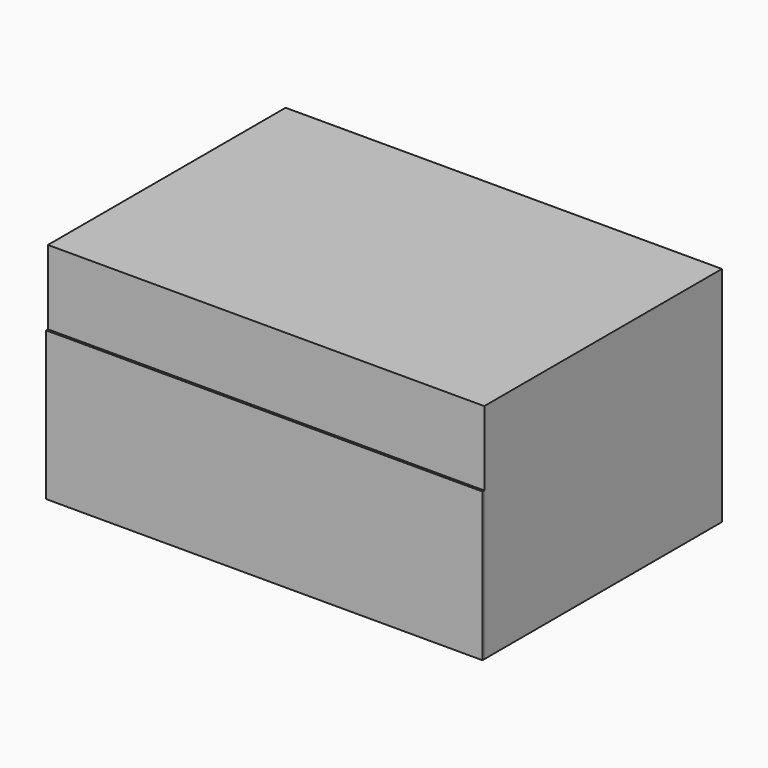
from build123d import *

# Parameters (mm, degrees)
F0_W     = 298.45
F0_H     = 152.4
F1_DEPTH = 101.6
F2_W     = 298.45
F2_H     = 101.6
F3_DEPTH = 1.5875


# Not quite as in the source:
# - a length typed as a fraction of an inch, garbled in the dataset ("3 / 203.2 mm" for 3/8 in), is restored


with BuildPart() as f1:
    # F0 (on Front) → F1 (new body, symmetric)
    with BuildSketch(Plane.XZ):
        Rectangle(F0_W, F0_H)
    extrude(amount=F1_DEPTH, both=True)


with BuildPart() as f3:
    # F2 (on face) → F3 (new body)
    with BuildSketch(Plane.XZ.offset(101.6)):
        with Locations((0, -25.4)):
            Rectangle(F2_W, F2_H)
    extrude(amount=F3_DEPTH)


solid = Compound([f1.part, f3.part])
